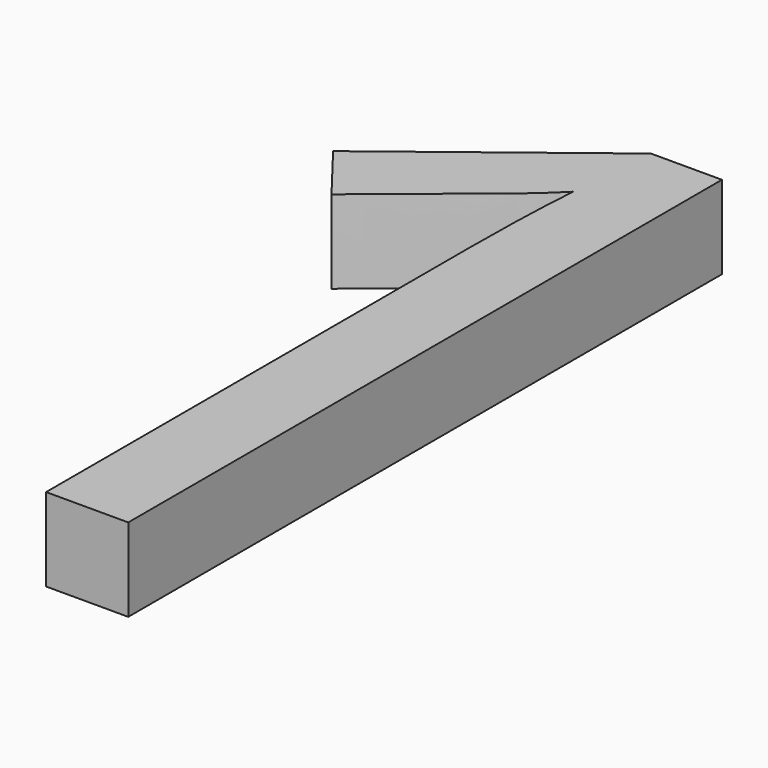
from build123d import *

# Parameters (mm, degrees)
F0_TEXT_SIZE = 12.5
F1_DEPTH     = 1


# Not quite as in the source:
# - Text() gives the source's letters only with a copy of the font that has no kerning and outlines rounded to 1/6400 em; it was checked with that copy


with BuildPart() as f1:
    # F0 (on Top) → F1 (new body)
    with BuildSketch(Plane.XY):
        with Locations((-35.5828859198, 17.8509426775)):
            Text('1', F0_TEXT_SIZE, font='Open Sans', text_align=(TextAlign.LEFT, TextAlign.BOTTOM))
    extrude(amount=F1_DEPTH)


solid = f1.part
